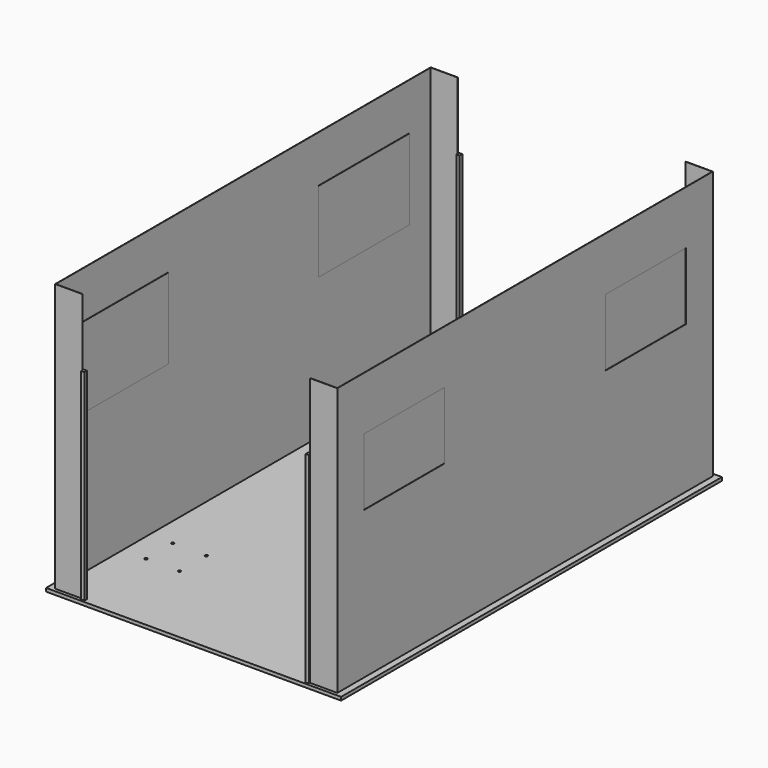
from build123d import *

# Parameters (mm, degrees)
F0_W      = 2200
F0_H      = 3500
F1_DEPTH  = 25
F2_W      = 500
F2_H      = 500
F3_DEPTH  = 25
F4_R      = 15
F5_DEPTH  = 50.001
F6_W      = 200
F6_H      = 200
F6_W_2    = 180
F6_H_2    = 180
F7_DEPTH  = 500
F8_W      = 350
F8_H      = 350
F9_DEPTH  = 25
F10_W     = 200
F10_H     = 2
F11_DEPTH = 2000
F13_W     = 750
F13_H     = 500
F14_DEPTH = 2
F12_W     = 750
F12_H     = 500
F15_DEPTH = 2
F16_W     = 850
F16_H     = 600
F16_W_2   = 750
F16_H_2   = 500
F17_DEPTH = 2
F18_W     = 850
F18_H     = 600
F18_W_2   = 750
F18_H_2   = 500
F19_DEPTH = 2
F20_R     = 10
F21_DEPTH = 25
F22_R     = 9
F23_DEPTH = 25
F24_DEPTH = 25
F25_DEPTH = 25
F27_DEPTH = 1500


with BuildPart() as f1:
    # F0 (on Top) → F1 (new body)
    with BuildSketch(Plane.XY):
        Rectangle(F0_W, F0_H)
    extrude(amount=F1_DEPTH)


with BuildPart() as f3:
    # F2 (on face) → F3 (new body)
    with BuildSketch(Plane.XY.offset(25)):
        Rectangle(F2_W, F2_H)
    extrude(amount=F3_DEPTH)


with BuildPart() as f5_tool:
    # F4 (on face) → F5 (new body, through all)
    with BuildSketch(Plane.XY.offset(50)):
        with Locations((-200, 200)):
            Circle(F4_R)
        with Locations((200, 200)):
            Circle(F4_R)
        with Locations((200, -200)):
            Circle(F4_R)
        with Locations((-200, -200)):
            Circle(F4_R)
    extrude(amount=-F5_DEPTH)


with BuildPart() as f1_1:
    add(f1.part)

    # F5: cut by f5_tool
    add(f5_tool.part, mode=Mode.SUBTRACT)

    # F20 (on face) → F21 (cut, through all)
    with BuildSketch(Plane.XY.offset(25)):
        with Locations((-625, 1125)):
            Circle(F20_R)
        with Locations((-875, 1125)):
            Circle(F20_R)
        with Locations((-625, 875)):
            Circle(F20_R)
        with Locations((-875, 875)):
            Circle(F20_R)
        with Locations((875, 875)):
            Circle(F20_R)
        with Locations((625, 875)):
            Circle(F20_R)
        with Locations((625, 1125)):
            Circle(F20_R)
        with Locations((875, 1125)):
            Circle(F20_R)
        with Locations((875, -1125)):
            Circle(F20_R)
        with Locations((-875, -875)):
            Circle(F20_R)
        with Locations((-625, -875)):
            Circle(F20_R)
        with Locations((-625, -1125)):
            Circle(F20_R)
        with Locations((-875, -1125)):
            Circle(F20_R)
        with Locations((875, -875)):
            Circle(F20_R)
        with Locations((625, -875)):
            Circle(F20_R)
        with Locations((625, -1125)):
            Circle(F20_R)
    extrude(amount=-F21_DEPTH, mode=Mode.SUBTRACT)

    # F24 (add): a face of the model
    f24_faces = [f1_1.faces().sort_by_distance(p)[0] for p in [
        (0, -1750, 12.5),
    ]]
    extrude(f24_faces, amount=F24_DEPTH)

    # F25 (add): a face of the model
    f25_faces = [f1_1.faces().sort_by_distance(p)[0] for p in [
        (0, 1750, 12.5),
    ]]
    extrude(f25_faces, amount=F25_DEPTH)


with BuildPart() as f3_1:
    add(f3.part)

    # F5: cut by f5_tool
    add(f5_tool.part, mode=Mode.SUBTRACT)

    # F6 (on face) → F7 (join)
    with BuildSketch(Plane.XY.offset(50)):
        Rectangle(F6_W, F6_H)
        Rectangle(F6_W_2, F6_H_2, mode=Mode.SUBTRACT)
    extrude(amount=F7_DEPTH)

    # F8 (on face) → F9 (join)
    with BuildSketch(Plane.XY.offset(550)):
        Rectangle(F8_W, F8_H)
    extrude(amount=F9_DEPTH)

    # F22 (on face) → F23 (cut, through all)
    with BuildSketch(Plane.XY.offset(575)):
        with Locations((-118, 122)):
            Circle(F22_R)
        with Locations((118, 122)):
            Circle(F22_R)
        with Locations((-118, -122)):
            Circle(F22_R)
        with Locations((118, -122)):
            Circle(F22_R)
    extrude(amount=-F23_DEPTH, mode=Mode.SUBTRACT)


with BuildPart() as f11:
    # F10 (on face) → F11 (new body)
    with BuildSketch(Plane.XY.offset(25)):
        with Locations((950, 1749)):
            Rectangle(F10_W, F10_H)
        Polygon((1052, 1750), (1050, 1750), (1050, 1748), (1050, -1748), (850, -1748), (850, -1750), (1050, -1750), (1052, -1750), align=None)
    extrude(amount=F11_DEPTH)

    # F12 (on face) → F15 (cut, through all)
    with BuildSketch(Plane.YZ.offset(1052)):
        with Locations((-1125, 1375)):
            Rectangle(F12_W, F12_H)
        with Locations((1125, 1375)):
            Rectangle(F12_W, F12_H)
    extrude(amount=-F15_DEPTH, mode=Mode.SUBTRACT)


with BuildPart() as f11b:
    # F10 (on face) → F11, piece 2 (new body)
    with BuildSketch(Plane.XY.offset(25)):
        with Locations((-950, 1749)):
            Rectangle(F10_W, F10_H)
        Polygon((-1050, 1748), (-1050, 1750), (-1052, 1750), (-1052, -1750), (-1050, -1750), (-850, -1750), (-850, -1748), (-1050, -1748), align=None)
    extrude(amount=F11_DEPTH)

    # F13 (on face) → F14 (cut, through all)
    with BuildSketch(Plane(origin=(-1052, 0, 0), x_dir=(0, -1, 0), z_dir=(-1, 0, 0))):
        with Locations((1125, 1375)):
            Rectangle(F13_W, F13_H)
        with Locations((-1125, 1375)):
            Rectangle(F13_W, F13_H)
    extrude(amount=-F14_DEPTH, mode=Mode.SUBTRACT)


with BuildPart() as f17:
    # F16 (on face) → F17 (new body)
    with BuildSketch(Plane.YZ.offset(-1050)):
        with Locations((-1125, 1375)):
            Rectangle(F16_W, F16_H)
        with Locations((-1125, 1375)):
            Rectangle(F16_W_2, F16_H_2, mode=Mode.SUBTRACT)
        with Locations((-1125, 1375)):
            Rectangle(F16_W_2, F16_H_2)
    extrude(amount=F17_DEPTH)


with BuildPart() as f17b:
    # F16 (on face) → F17, piece 2 (new body)
    with BuildSketch(Plane.YZ.offset(-1050)):
        with Locations((1125, 1375)):
            Rectangle(F16_W, F16_H)
        with Locations((1125, 1375)):
            Rectangle(F16_W_2, F16_H_2, mode=Mode.SUBTRACT)
        with Locations((1125, 1375)):
            Rectangle(F16_W_2, F16_H_2)
    extrude(amount=F17_DEPTH)


with BuildPart() as f19:
    # F18 (on face) → F19 (new body)
    with BuildSketch(Plane(origin=(1050, 0, 0), x_dir=(0, -1, 0), z_dir=(-1, 0, 0))):
        with Locations((-1125, 1375)):
            Rectangle(F18_W, F18_H)
        with Locations((-1125, 1375)):
            Rectangle(F18_W_2, F18_H_2, mode=Mode.SUBTRACT)
        with Locations((-1125, 1375)):
            Rectangle(F18_W_2, F18_H_2)
    extrude(amount=F19_DEPTH)


with BuildPart() as f19b:
    # F18 (on face) → F19, piece 2 (new body)
    with BuildSketch(Plane(origin=(1050, 0, 0), x_dir=(0, -1, 0), z_dir=(-1, 0, 0))):
        with Locations((1125, 1375)):
            Rectangle(F18_W, F18_H)
        with Locations((1125, 1375)):
            Rectangle(F18_W_2, F18_H_2, mode=Mode.SUBTRACT)
        with Locations((1125, 1375)):
            Rectangle(F18_W_2, F18_H_2)
    extrude(amount=F19_DEPTH)


with BuildPart() as f27:
    # F26 (on face) → F27 (new body)
    with BuildSketch(Plane.XY.offset(25)):
        Polygon((850, 1749), (850, 1750), (850, 1761.5), (825, 1761.5), (825, 1736.5), (850, 1736.5), (850, 1748), align=None)
    extrude(amount=F27_DEPTH)


with BuildPart() as f27b:
    # F26 (on face) → F27, piece 2 (new body)
    with BuildSketch(Plane.XY.offset(25)):
        Polygon((-850, 1761.5), (-850, 1750), (-850, 1749), (-850, 1748), (-850, 1736.5), (-825, 1736.5), (-825, 1749), (-825, 1761.5), align=None)
    extrude(amount=F27_DEPTH)


with BuildPart() as f27c:
    # F26 (on face) → F27, piece 3 (new body)
    with BuildSketch(Plane.XY.offset(25)):
        Polygon((-850, -1749), (-850, -1750), (-850, -1761.5), (-825, -1761.5), (-825, -1749), (-825, -1736.5), (-850, -1736.5), (-850, -1748), align=None)
    extrude(amount=F27_DEPTH)


with BuildPart() as f27d:
    # F26 (on face) → F27, piece 4 (new body)
    with BuildSketch(Plane.XY.offset(25)):
        Polygon((850, -1750), (850, -1749), (850, -1748), (850, -1736.5), (825, -1736.5), (825, -1761.5), (850, -1761.5), align=None)
    extrude(amount=F27_DEPTH)


solid = Compound([f1_1.part, f3_1.part, f11.part, f11b.part, f17.part, f17b.part, f19.part, f19b.part, f27.part, f27b.part, f27c.part, f27d.part])
